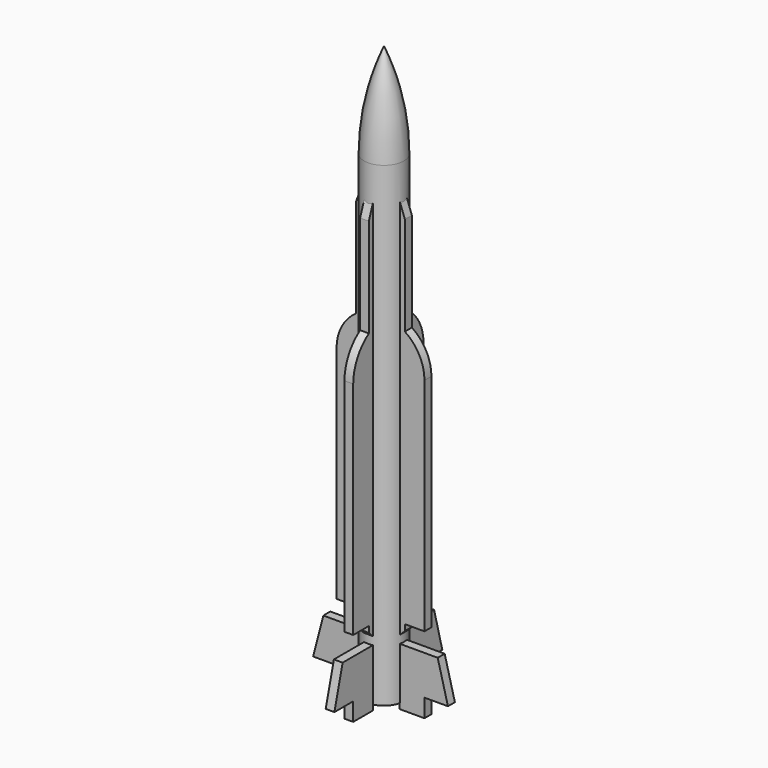
from build123d import *

# Parameters (mm, degrees)
F2_W     = 0.8680555556
F2_H     = 1.6279645497
F3_DEPTH = 0.2
F4_COUNT = 4


# Not quite as in the source:
# - a feature names something its author has since deleted; it is built from what else it names


with BuildPart() as f1:
    # F0 (on Front) → F1 (revolve)
    with BuildSketch(Plane.XZ):
        with BuildLine():
            Line((0, 26.1458333333), (0, 0))
            Line((0, 0), (0.9097222222, 0))
            Line((0.9097222222, 0), (0.9097222222, 21.8055555556))
            ThreePointArc((0.9097222222, 21.8055555556), (0.6798471947, 24.0228515276), (0, 26.1458333333))
        make_face()
    revolve(axis=Axis((0, 0, 13.0729166667), (0, 0, 1)))

    # F2 (on Front) → F3 (join, symmetric)
    with BuildSketch(Plane.XZ):
        with Locations((0.4340277778, 0.8139822748)):
            Rectangle(F2_W, F2_H)
        with BuildLine():
            Line((0, 22.6730523746), (0, 1.6279645497))
            Line((0, 1.6279645497), (0.8680555556, 1.6279645497))
            Line((0.8680555556, 1.6279645497), (0.8680555556, 0))
            Line((0.8680555556, 0), (0.8680555556, -0.2430555556))
            Line((0.8680555556, -0.2430555556), (2.0138888889, -0.2430555556))
            Line((2.0138888889, -0.2430555556), (2.0138888889, 0.5902777778))
            Line((2.0138888889, 0.5902777778), (3.0902777778, 0.5902777778))
            Line((3.0902777778, 0.5902777778), (2.6215277778, 2.3958333333))
            Line((2.6215277778, 2.3958333333), (0.8, 2.3958333333))
            Line((0.8, 2.3958333333), (0.8, 2.6680555556))
            Line((0.8, 2.6680555556), (1.1180555556, 2.9861111111))
            Line((1.1180555556, 2.9861111111), (1.1180555556, 3.2638888889))
            Line((1.1180555556, 3.2638888889), (2.0138888889, 3.2638888889))
            Line((2.0138888889, 3.2638888889), (2.0138888889, 13.3944219874))
            ThreePointArc((2.0138888889, 13.3944219874), (1.7758643131, 14.3441874312), (1.1180555556, 15.0694444444))
            Line((1.1180555556, 15.0694444444), (1.1180555556, 19.6012199821))
            Line((1.1180555556, 19.6012199821), (0, 22.6730523746))
        make_face()
    extrude(amount=F3_DEPTH, both=True)

    # F4: F1 ×4 about axis
    f4_axis = Axis((0, 0, 0), (0, 0, 1))


with BuildPart() as f1_1:
    add(f1.part)
    for i in range(1, F4_COUNT):
        add(f1.part.rotate(f4_axis, i * 360 / F4_COUNT))


solid = f1_1.part
